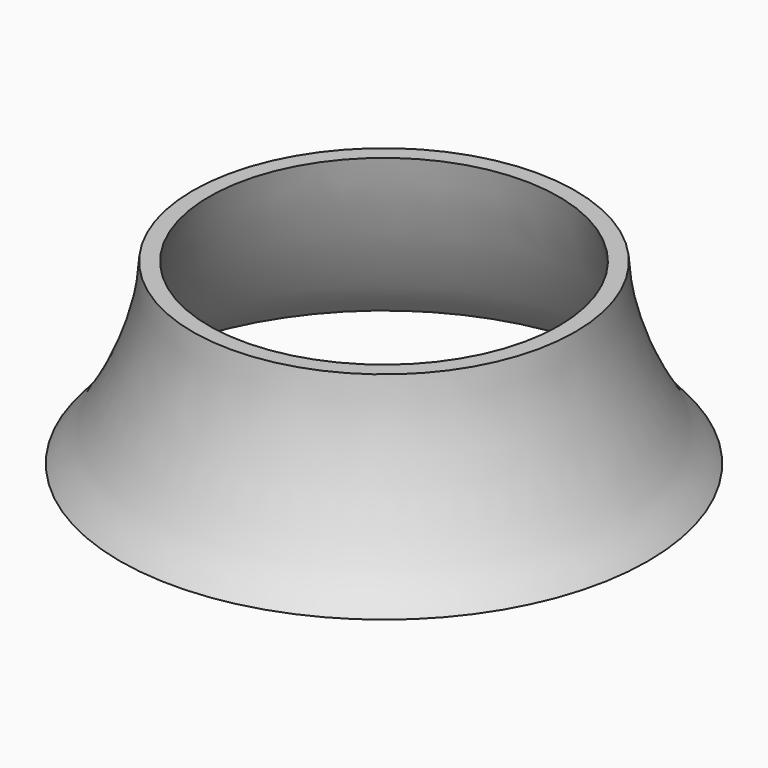
from build123d import *


with BuildPart() as f4:
    # F4: sweep along a path in F2
    with BuildLine(Plane.XY.offset(16.29)) as f4_path:
        CenterArc((0, 0), 17.5, 0, 360)
    # F3 (on Front) → F4 (sweep)
    with BuildSketch(Plane.XZ):
        with BuildLine():
            add(Edge.make_bspline(
                [(-24.165, 0), (-22.7628440457, 1.6847910613), (-22.2386035811, 2.0176427038), (-17.800130412, 10.0504284315), (-17.5, 16.29)],
                knots=[0, 0, 0, 0, 0.3316460871, 1, 1, 1, 1], degree=3))
            Line((-24.165, 0), (-23.665, 0))
            add(Edge.make_bspline(
                [(-23.665, 0), (-22.2955542786, 1.5072109543), (-21.6855979109, 2.0542739255), (-17.1840847583, 10.0504284315), (-16, 16.29)],
                knots=[0, 0, 0, 0, 0.325916747, 1, 1, 1, 1], degree=3))
            Line((-16, 16.29), (-17.5, 16.29))
        make_face()
    sweep(path=f4_path.line)


solid = f4.part
